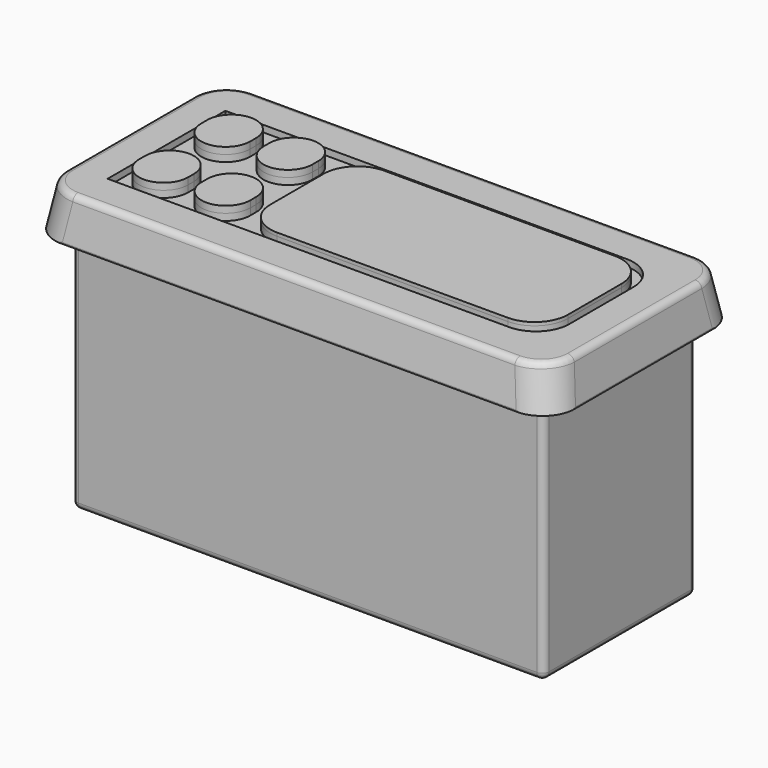
from build123d import *

# Parameters (mm, degrees)
F0_W         = 77.65
F0_H         = 35.4
F1_DEPTH     = 6.3
F2_W         = 70.5
F2_H         = 28.5
F3_DEPTH     = 36.6
F4_W         = 19.2
F4_H         = 15.5
F5_DEPTH     = 2
F6_DEPTH     = 12
F7_W         = 65
F7_H         = 22
F7_W_2       = 44.5
F7_H_2       = 20
F8_DEPTH     = 1
F9_DEPTH     = 1
F10_DEPTH    = 0.5
F11_SIZE2    = 6.1
F11_SIZE     = 1
F12_T1_DEPTH = 54.9699145881
F12_T3_DEPTH = 54.9699145881
F12_T5_DEPTH = 54.9699145881
F12_T7_DEPTH = 54.9699145881
F13_R        = 1
F14_R        = 5
F14_2_R      = 5


# Not quite as in the source:
# - a fillet or chamfer that OpenCascade refuses, or shapes differently, is made with other operations: its cross-section is extruded or revolved along the edge and cut away or added


with BuildPart() as f1:
    # F0 (on Top) → F1 (new body)
    with BuildSketch(Plane.XY):
        with Locations((38.825, 17.7)):
            Rectangle(F0_W, F0_H)
    extrude(amount=F1_DEPTH)

    # F2 (on face) → F3 (join)
    with BuildSketch(Plane(origin=(0, 0, 0), x_dir=(1, 0, 0), z_dir=(0, 0, -1))):
        with Locations((38.825, -17.7)):
            Rectangle(F2_W, F2_H)
    extrude(amount=F3_DEPTH)

    # F4 (on face) → F5 (join)
    with BuildSketch(Plane(origin=(0, 0, -36.6), x_dir=(1, 0, 0), z_dir=(0, 0, -1))):
        with Locations((38.825, -21.2)):
            Rectangle(F4_W, F4_H)
        Polygon((45.075, -17.45), (45.075, -24.95), (41.975, -24.95), (41.975, -27.95), (35.675, -27.95), (35.675, -24.95), (32.575, -24.95), (32.575, -17.45), align=None, mode=Mode.SUBTRACT)
    extrude(amount=F5_DEPTH)

    # F6 (cut): a face of the model
    f6_faces = [f1.faces().sort_by_distance(p)[0] for p in [
        (38.825, 22.0808255659, -36.6),
    ]]
    extrude(f6_faces, amount=-F6_DEPTH, mode=Mode.SUBTRACT)

    # F7 (on face) → F8 (cut)
    with BuildSketch(Plane.XY.offset(6.3)):
        with Locations((38.825, 17.7)):
            Rectangle(F7_W, F7_H)
        with BuildLine():
            ThreePointArc((14.625, 11.35), (10.975, 7.7), (7.325, 11.35))
            Line((7.325, 11.35), (7.325, 11.9))
            Line((7.325, 11.9), (7.325, 12.45))
            ThreePointArc((7.325, 12.45), (10.975, 16.1), (14.625, 12.45))
            Line((14.625, 12.45), (14.625, 11.9))
            Line((14.625, 11.9), (14.625, 11.35))
        make_face(mode=Mode.SUBTRACT)
        with BuildLine():
            ThreePointArc((16.625, 12.45), (20.275, 16.1), (23.925, 12.45))
            Line((23.925, 12.45), (23.925, 11.9))
            Line((23.925, 11.9), (23.925, 11.35))
            ThreePointArc((23.925, 11.35), (20.275, 7.7), (16.625, 11.35))
            Line((16.625, 11.35), (16.625, 11.9))
            Line((16.625, 11.9), (16.625, 12.45))
        make_face(mode=Mode.SUBTRACT)
        with BuildLine():
            Line((7.325, 23.5), (7.325, 24.05))
            ThreePointArc((7.325, 24.05), (10.975, 27.7), (14.625, 24.05))
            Line((14.625, 24.05), (14.625, 23.5))
            Line((14.625, 23.5), (14.625, 22.95))
            ThreePointArc((14.625, 22.95), (10.975, 19.3), (7.325, 22.95))
            Line((7.325, 22.95), (7.325, 23.5))
        make_face(mode=Mode.SUBTRACT)
        with BuildLine():
            ThreePointArc((16.625, 24.05), (20.275, 27.7), (23.925, 24.05))
            Line((23.925, 24.05), (23.925, 23.5))
            Line((23.925, 23.5), (23.925, 22.95))
            ThreePointArc((23.925, 22.95), (20.275, 19.3), (16.625, 22.95))
            Line((16.625, 22.95), (16.625, 23.5))
            Line((16.625, 23.5), (16.625, 24.05))
        make_face(mode=Mode.SUBTRACT)
        with Locations((48.075, 17.7)):
            Rectangle(F7_W_2, F7_H_2, mode=Mode.SUBTRACT)
    extrude(amount=-F8_DEPTH, mode=Mode.SUBTRACT)


with BuildPart() as f9:
    # F9 (new): a face of the model
    f9_faces = [f1.part.faces().sort_by_distance(p)[0] for p in [
        (20.275, 11.9, 6.3),
    ]]
    extrude(f9_faces, amount=F9_DEPTH)


with BuildPart() as f9b:
    # F9#2 (new): a face of the model
    f9_2_faces = [f1.part.faces().sort_by_distance(p)[0] for p in [
        (10.975, 11.9, 6.3),
    ]]
    extrude(f9_2_faces, amount=F9_DEPTH)


with BuildPart() as f9c:
    # F9#3 (new): a face of the model
    f9_3_faces = [f1.part.faces().sort_by_distance(p)[0] for p in [
        (10.975, 23.5, 6.3),
    ]]
    extrude(f9_3_faces, amount=F9_DEPTH)


with BuildPart() as f9d:
    # F9#4 (new): a face of the model
    f9_4_faces = [f1.part.faces().sort_by_distance(p)[0] for p in [
        (20.275, 23.5, 6.3),
    ]]
    extrude(f9_4_faces, amount=F9_DEPTH)


with BuildPart() as f10:
    # F10 (new): a face of the model
    f10_faces = [f1.part.faces().sort_by_distance(p)[0] for p in [
        (48.075, 17.7, 6.3),
    ]]
    extrude(f10_faces, amount=F10_DEPTH)

    # F14#2
    f14_2_edges = [f10.edges().sort_by_distance(p)[0] for p in [
        (25.825, 7.7, 6.55),
        (25.825, 27.7, 6.55),
        (70.325, 27.7, 6.55),
        (70.325, 7.7, 6.55),
    ]]
    fillet(f14_2_edges, radius=F14_2_R)


with BuildPart() as f1_1:
    add(f1.part)

    # F11
    f11_edges = [f1_1.edges().sort_by_distance(p)[0] for p in [
        (77.65, 17.7, 6.3),
        (38.825, 35.4, 6.3),
        (0, 17.7, 6.3),
        (38.825, 0, 6.3),
    ]]
    f11_side = f1_1.faces().sort_by_distance((0.853386, 17.7, 6.3))[0]
    chamfer(f11_edges, length=F11_SIZE, length2=F11_SIZE2, reference=f11_side)

    # F12: fillet of radius 5 on 4 edges, made by hand

    # F12_s2 → F12_t1 (cut)
    with BuildSketch(Plane(origin=(2.9757714869, 2.9757714869, 18.1522060699), x_dir=(0.7071067812, -0.7071067812, 0), z_dir=(-0.1596987728, -0.1596987728, -0.9741625141))):
        with BuildLine():
            ThreePointArc((-3.4889626693, -3.3536470115), (0, -1.9351466265), (3.4889626693, -3.3536470115))
            Line((3.4889626693, -3.3536470115), (0, 0.0451696341))
            Line((0, 0.0451696341), (-3.4889626693, -3.3536470115))
        make_face()
    extrude(amount=F12_T1_DEPTH, mode=Mode.SUBTRACT)

    # F12_s4 → F12_t3 (cut)
    with BuildSketch(Plane(origin=(-0.9954093344, 0.9954093344, 6.0719969396), x_dir=(0.7071067812, 0.7071067812, 0), z_dir=(0.1596987728, -0.1596987728, -0.9741625141))):
        with BuildLine():
            ThreePointArc((51.4178788898, 50.1345398044), (54.9068415591, 51.5530401894), (58.3958042284, 50.1345398044))
            Line((58.3958042284, 50.1345398044), (54.9068415591, 53.53335645))
            Line((54.9068415591, 53.53335645), (51.4178788898, 50.1345398044))
        make_face()
    extrude(amount=F12_T3_DEPTH, mode=Mode.SUBTRACT)

    # F12_s6 → F12_t5 (cut)
    with BuildSketch(Plane(origin=(-0.0925784239, -0.0925784239, 0.5647283856), x_dir=(-0.7071067812, 0.7071067812, 0), z_dir=(0.1596987728, 0.1596987728, -0.9741625141))):
        with BuildLine():
            ThreePointArc((-26.3862988358, 74.5193667624), (-29.8752615051, 75.9378671474), (-33.3642241744, 74.5193667624))
            Line((-33.3642241744, 74.5193667624), (-29.8752615051, 77.918183408))
            Line((-29.8752615051, 77.918183408), (-26.3862988358, 74.5193667624))
        make_face()
    extrude(amount=F12_T5_DEPTH, mode=Mode.SUBTRACT)

    # F12_s8 → F12_t7 (cut)
    with BuildSketch(Plane(origin=(2.0729405764, -2.0729405764, 12.6449375159), x_dir=(-0.7071067812, -0.7071067812, 0), z_dir=(-0.1596987728, 0.1596987728, -0.9741625141))):
        with BuildLine():
            ThreePointArc((-21.5426173847, 21.0311799464), (-25.031580054, 22.4496803314), (-28.5205427233, 21.0311799464))
            Line((-28.5205427233, 21.0311799464), (-25.031580054, 24.429996592))
            Line((-25.031580054, 24.429996592), (-21.5426173847, 21.0311799464))
        make_face()
    extrude(amount=F12_T7_DEPTH, mode=Mode.SUBTRACT)

    # F13
    f13_edges = [f1_1.edges().sort_by_distance(p)[0] for p in [
        (38.825, 34.4, 6.3),
        (3.575, 3.45, -18.3),
        (3.575, 31.95, -18.3),
        (74.075, 31.95, -18.3),
        (74.075, 3.45, -18.3),
        (74.075, 17.7, -36.6),
        (38.825, 3.45, -36.6),
        (3.575, 17.7, -36.6),
        (38.825, 31.95, -36.6),
    ]]
    fillet(f13_edges, radius=F13_R)

    # F14
    f14_edges = [f1_1.edges().sort_by_distance(p)[0] for p in [
        (25.825, 7.7, 5.8),
        (25.825, 27.7, 5.8),
        (70.325, 27.7, 5.8),
        (70.325, 7.7, 5.8),
        (71.325, 6.7, 5.8),
        (71.325, 28.7, 5.8),
    ]]
    fillet(f14_edges, radius=F14_R)


solid = Compound([f9.part, f9b.part, f9c.part, f9d.part, f10.part, f1_1.part])
